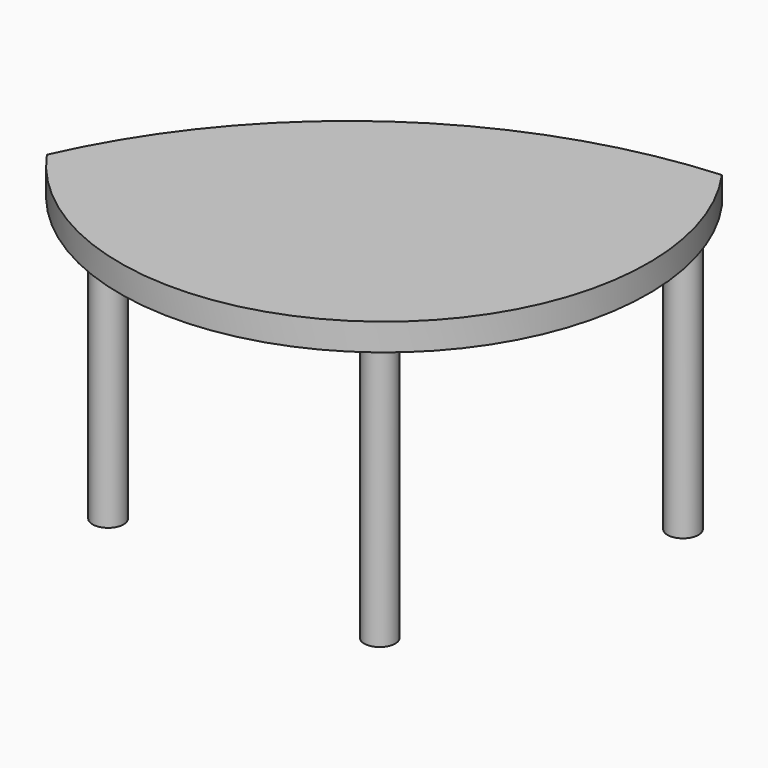
from build123d import *

# Parameters (mm, degrees)
F0_R     = 22.9132131763
F1_DEPTH = 40
F2_DEPTH = 400


# Not quite as in the source:
# - a feature names something its author has since deleted; it is built from what else it names


with BuildPart() as f1:
    # F0 (on Top) → F1 (new body)
    with BuildSketch(Plane.XY):
        with BuildLine():
            ThreePointArc((-599.9922642108, -94.5975626578), (-55.9908868153, -192.3217779419), (39.4396888844, 352.0866405113))
            ThreePointArc((39.4396888844, 352.0866405113), (-342.3269144878, 217.5704996833), (-599.9922642108, -94.5975626578))
        make_face()
        with Locations((-505.0551273235, -100.2501100564)):
            Circle(F0_R, mode=Mode.SUBTRACT)
        with Locations((-74.5249837637, -137.0074301958)):
            Circle(F0_R, mode=Mode.SUBTRACT)
        with Locations((28.9413593709, 293.3445572853)):
            Circle(F0_R, mode=Mode.SUBTRACT)
        with Locations((28.9413593709, 293.3445572853)):
            Circle(F0_R)
        with Locations((-74.5249837637, -137.0074301958)):
            Circle(F0_R)
        with Locations((-505.0551273235, -100.2501100564)):
            Circle(F0_R)
    extrude(amount=F1_DEPTH)

    # F0 (on Top) → F2 (join)
    with BuildSketch(Plane.XY):
        with Locations((-505.0551273235, -100.2501100564)):
            Circle(F0_R)
        with Locations((-74.5249837637, -137.0074301958)):
            Circle(F0_R)
        with Locations((28.9413593709, 293.3445572853)):
            Circle(F0_R)
    extrude(amount=-F2_DEPTH)


solid = f1.part
